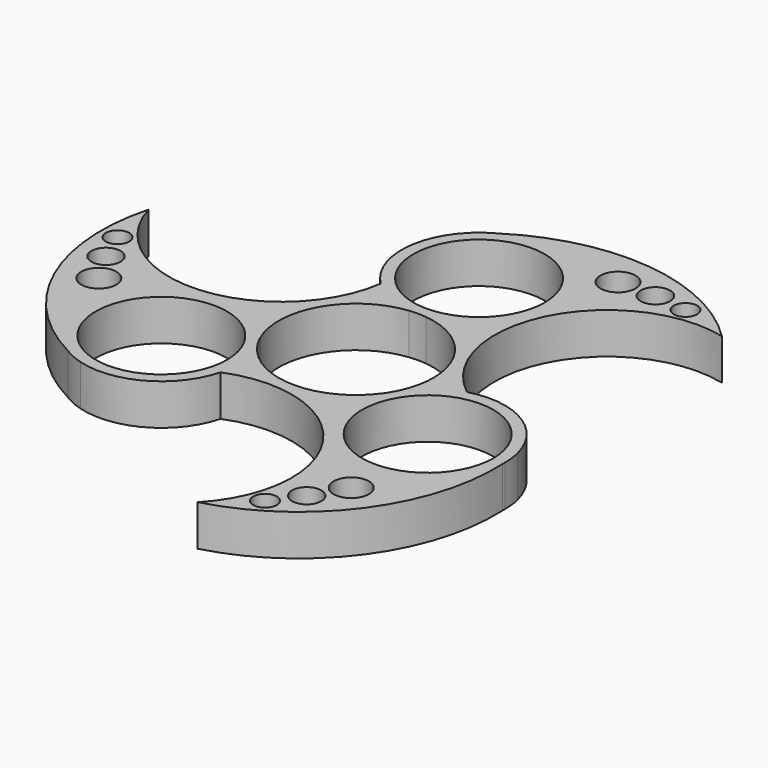
from build123d import *

# Parameters (mm, degrees)
F0_R     = 11.2
F0_R_2   = 3
F0_R_3   = 2.5
F0_R_4   = 2
F1_DEPTH = 7


# Not quite as in the source:
# - a feature names something its author has since deleted; it is built from what else it names


with BuildPart() as f1:
    # F0 (on Top) → F1 (new body)
    with BuildSketch(Plane.XY):
        with BuildLine():
            ThreePointArc((-6.1736201838, 37.9133765769), (-7.7319005407, 36.9445453014), (-9.1407759551, 35.7689851037))
            ThreePointArc((-9.1407759551, 35.7689851037), (-7.6864399565, 36.8816423115), (-6.1736201838, 37.9133765769))
        make_face()
        with BuildLine():
            ThreePointArc((-26.4064617899, -25.8006367392), (-28.0972191968, -25.0974734227), (-29.7471371669, -24.3032002009))
            ThreePointArc((-29.7471371669, -24.3032002009), (-28.1289644919, -25.1682949385), (-26.4064617899, -25.8006367392))
        make_face()
        with BuildLine():
            ThreePointArc((35.929749598, -13.123027049), (35.8337727119, -11.5341349098), (35.5472377449, -9.9683483645))
            ThreePointArc((35.5472377449, -9.9683483645), (35.7836591533, -11.7841688888), (35.9207573507, -13.610176376))
            ThreePointArc((35.9207573507, -13.610176376), (35.9275013447, -13.3666432057), (35.929749598, -13.123027049))
        make_face()
        with BuildLine():
            ThreePointArc((-6.1736201838, 37.9133765769), (-7.6864399565, 36.8816423115), (-9.1407759551, 35.7689851037))
            ThreePointArc((-9.1407759551, 35.7689851037), (-13.1996365954, 26.3440017791), (-9.2810910796, 16.8598222464))
            ThreePointArc((-9.2810910796, 16.8598222464), (-5.669005002, 14.3253837189), (-1.4234328474, 13.123027049))
            ThreePointArc((-1.4234328474, 13.123027049), (0, 13.2), (1.4234328474, 13.123027049))
            ThreePointArc((1.4234328474, 13.123027049), (9.824187335, 17.4298563231), (13.2, 26.246054098))
            ThreePointArc((13.2, 26.246054098), (6.8098536539, 37.5538343052), (-6.1736201838, 37.9133765769))
        make_face()
        with Locations((0, 26.246054098)):
            Circle(F0_R, mode=Mode.SUBTRACT)
        with BuildLine():
            ThreePointArc((-10.6531583753, -7.7942425309), (-11.43153533, -6.6), (-12.0765912227, -5.3287845181))
            ThreePointArc((-12.0765912227, -5.3287845181), (-32.389553942, -4.1270179319), (-29.7471371669, -24.3032002009))
            ThreePointArc((-29.7471371669, -24.3032002009), (-28.0972191968, -25.0974734227), (-26.4064617899, -25.8006367392))
            ThreePointArc((-26.4064617899, -25.8006367392), (-16.2147564803, -24.6032215019), (-9.9604888289, -16.467571773))
            ThreePointArc((-9.9604888289, -16.467571773), (-9.6378772691, -14.8091109508), (-9.529749598, -13.123027049))
            ThreePointArc((-9.529749598, -13.123027049), (-9.8136549069, -10.4000694786), (-10.6531583753, -7.7942425309))
        make_face()
        with Locations((-22.729749598, -13.123027049)):
            Circle(F0_R, mode=Mode.SUBTRACT)
        with BuildLine():
            ThreePointArc((35.5472377449, -9.9683483645), (29.4143930758, -1.7407802772), (19.2415799085, -0.3922504734))
            ThreePointArc((19.2415799085, -0.3922504734), (15.2406487206, -2.2531895135), (12.0765912227, -5.3287845181))
            ThreePointArc((12.0765912227, -5.3287845181), (11.43153533, -6.6), (10.6531583753, -7.7942425309))
            ThreePointArc((10.6531583753, -7.7942425309), (19.7688793419, -25.9866675651), (35.9207573507, -13.610176376))
            ThreePointArc((35.9207573507, -13.610176376), (35.7836591533, -11.7841688888), (35.5472377449, -9.9683483645))
        make_face()
        with Locations((22.729749598, -13.123027049)):
            Circle(F0_R, mode=Mode.SUBTRACT)
        with BuildLine():
            ThreePointArc((-1.4234328474, 13.123027049), (-5.669005002, 14.3253837189), (-9.2810910796, 16.8598222464))
            ThreePointArc((-9.2810910796, 16.8598222464), (-26.9770057804, 0.3443606169), (-46.801379663, 14.2332075847))
            ThreePointArc((-46.801379663, 14.2332075847), (-45.0709674202, -8.0428719823), (-29.7471371669, -24.3032002009))
            ThreePointArc((-29.7471371669, -24.3032002009), (-32.389553942, -4.1270179319), (-12.0765912227, -5.3287845181))
            ThreePointArc((-12.0765912227, -5.3287845181), (-11.43153533, 6.6), (-1.4234328474, 13.123027049))
        make_face()
        with Locations((-39.597851646, -5.3848865237)):
            Circle(F0_R_2, mode=Mode.SUBTRACT)
        with Locations((-42.7842679926, 0.1341484827)):
            Circle(F0_R_3, mode=Mode.SUBTRACT)
        with Locations((-45.0379561931, 5.4032604173)):
            Circle(F0_R_4, mode=Mode.SUBTRACT)
        with BuildLine():
            ThreePointArc((35.7270091772, 33.4145799279), (15.570152254, 43.0540387502), (-6.1736201838, 37.9133765769))
            ThreePointArc((-6.1736201838, 37.9133765769), (6.8098536539, 37.5538343052), (13.2, 26.246054098))
            ThreePointArc((13.2, 26.246054098), (9.824187335, 17.4298563231), (1.4234328474, 13.123027049))
            ThreePointArc((1.4234328474, 13.123027049), (9.824187335, 8.816197775), (13.2, 0))
            ThreePointArc((13.2, 0), (12.9160946911, -2.7229575704), (12.0765912227, -5.3287845181))
            ThreePointArc((12.0765912227, -5.3287845181), (15.2406487206, -2.2531895135), (19.2415799085, -0.3922504734))
            ThreePointArc((19.2415799085, -0.3922504734), (13.7867279325, 23.1905920154), (35.7270091772, 33.4145799279))
        make_face()
        with Locations((15.135477297, 36.9851887226)):
            Circle(F0_R_2, mode=Mode.SUBTRACT)
        with Locations((21.5083099902, 36.9851887226)):
            Circle(F0_R_3, mode=Mode.SUBTRACT)
        with Locations((27.1983388811, 36.3023839891)):
            Circle(F0_R_4, mode=Mode.SUBTRACT)
        with BuildLine():
            ThreePointArc((10.6531583753, -7.7942425309), (0, -13.2), (-10.6531583753, -7.7942425309))
            ThreePointArc((-10.6531583753, -7.7942425309), (-9.8136549069, -10.4000694786), (-9.529749598, -13.123027049))
            ThreePointArc((-9.529749598, -13.123027049), (-9.6378772691, -14.8091109508), (-9.9604888289, -16.467571773))
            ThreePointArc((-9.9604888289, -16.467571773), (13.1902778479, -23.5349526323), (11.0743704858, -47.6477875127))
            ThreePointArc((11.0743704858, -47.6477875127), (29.5008151662, -35.0111667679), (35.9207573507, -13.610176376))
            ThreePointArc((35.9207573507, -13.610176376), (19.7688793419, -25.9866675651), (10.6531583753, -7.7942425309))
        make_face()
        with Locations((17.8396173119, -41.7056444063)):
            Circle(F0_R_4, mode=Mode.SUBTRACT)
        with Locations((21.2759580025, -37.1193372053)):
            Circle(F0_R_3, mode=Mode.SUBTRACT)
        with Locations((24.462374349, -31.6003021989)):
            Circle(F0_R_2, mode=Mode.SUBTRACT)
    extrude(amount=F1_DEPTH)


solid = f1.part
